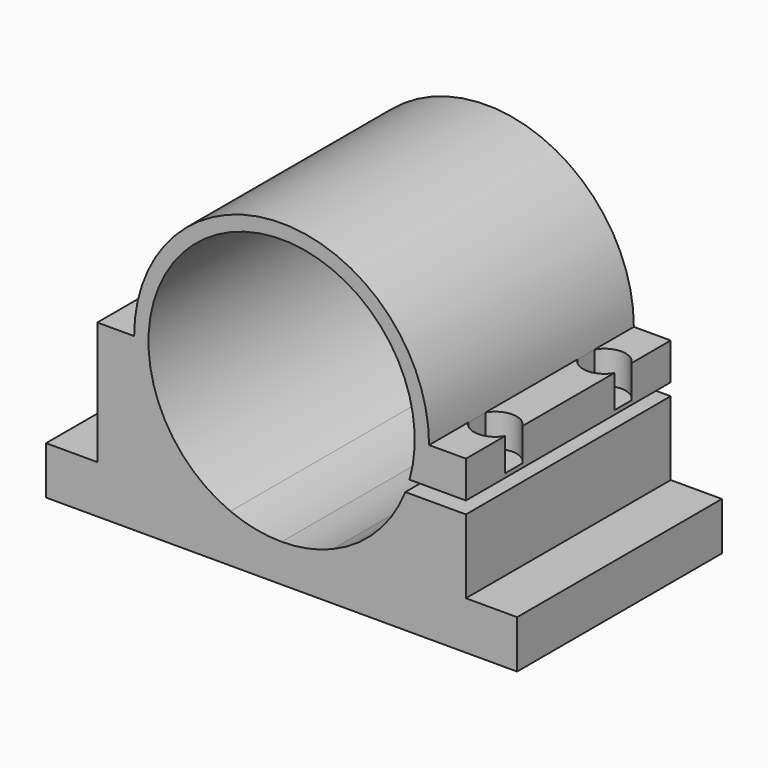
from build123d import *

# Parameters (mm, degrees)
F0_W     = 146.05
F0_H     = 79.375
F1_DEPTH = 14.859
F3_DEPTH = 79.375
F4_DEPTH = 85.725
F6_DEPTH = 79.376
F8_DEPTH = 10.16


with BuildPart() as f1:
    # F0 (on Top) → F1 (new body)
    with BuildSketch(Plane.XY):
        Rectangle(F0_W, F0_H)
    extrude(amount=F1_DEPTH)

    # F2 (on face) → F3 (join)
    with BuildSketch(Plane.XZ.offset(39.6875)):
        with BuildLine():
            Line((-57.15, 14.859), (-15.875, 14.859))
            ThreePointArc((-15.875, 14.859), (-22.8952505992, 87.3018758988), (41.275, 52.959))
            ThreePointArc((41.275, 52.959), (34.3428758988, 30.0637494008), (15.875, 14.859))
            Line((15.875, 14.859), (57.15, 14.859))
            Line((57.15, 14.859), (57.15, 52.959))
            Line((57.15, 52.959), (45.72, 52.959))
            ThreePointArc((45.72, 52.959), (0, 98.679), (-45.72, 52.959))
            Line((-45.72, 52.959), (-57.15, 52.959))
            Line((-57.15, 52.959), (-57.15, 14.859))
        make_face()
    extrude(amount=-F3_DEPTH)

    # F2 (on face) → F4 (cut)
    with BuildSketch(Plane.XZ.offset(39.6875)):
        with BuildLine():
            Line((0, 14.859), (0, 11.684))
            ThreePointArc((0, 11.684), (8.0946934778, 12.4855326109), (15.875, 14.859))
            Line((15.875, 14.859), (0, 14.859))
        make_face()
        with BuildLine():
            ThreePointArc((-15.875, 14.859), (-8.0946934778, 12.4855326109), (0, 11.684))
            Line((0, 11.684), (0, 14.859))
            Line((0, 14.859), (-15.875, 14.859))
        make_face()
    extrude(amount=-F4_DEPTH, mode=Mode.SUBTRACT)

    # F5 (on face) → F6 (cut, through all)
    with BuildSketch(Plane.XZ.offset(39.6875)):
        with BuildLine():
            Line((57.15, 37.7415791154), (57.15, 41.5375120938))
            Line((57.15, 41.5375120938), (39.6632731757, 41.5375120938))
            ThreePointArc((39.6632731757, 41.5375120938), (39.0614634109, 39.6237946698), (38.3673784174, 37.7415791154))
            Line((38.3673784174, 37.7415791154), (57.15, 37.7415791154))
        make_face()
    extrude(amount=-F6_DEPTH, mode=Mode.SUBTRACT)

    # F7 (on face) → F8 (cut)
    with BuildSketch(Plane.XY.offset(52.959)):
        with BuildLine():
            Line((57.15, 17.8361811879), (57.15, 24.4548188121))
            ThreePointArc((57.15, 24.4548188121), (51.435, 27.7495), (45.72, 24.4548188121))
            Line((45.72, 24.4548188121), (45.72, 17.8361811879))
            ThreePointArc((45.72, 17.8361811879), (51.435, 14.5415), (57.15, 17.8361811879))
        make_face()
        with BuildLine():
            Line((57.15, -24.4548188121), (57.15, -17.8361811879))
            ThreePointArc((57.15, -17.8361811879), (51.435, -14.5415), (45.72, -17.8361811879))
            Line((45.72, -17.8361811879), (45.72, -24.4548188121))
            ThreePointArc((45.72, -24.4548188121), (51.435, -27.7495), (57.15, -24.4548188121))
        make_face()
    extrude(amount=-F8_DEPTH, mode=Mode.SUBTRACT)


solid = f1.part
